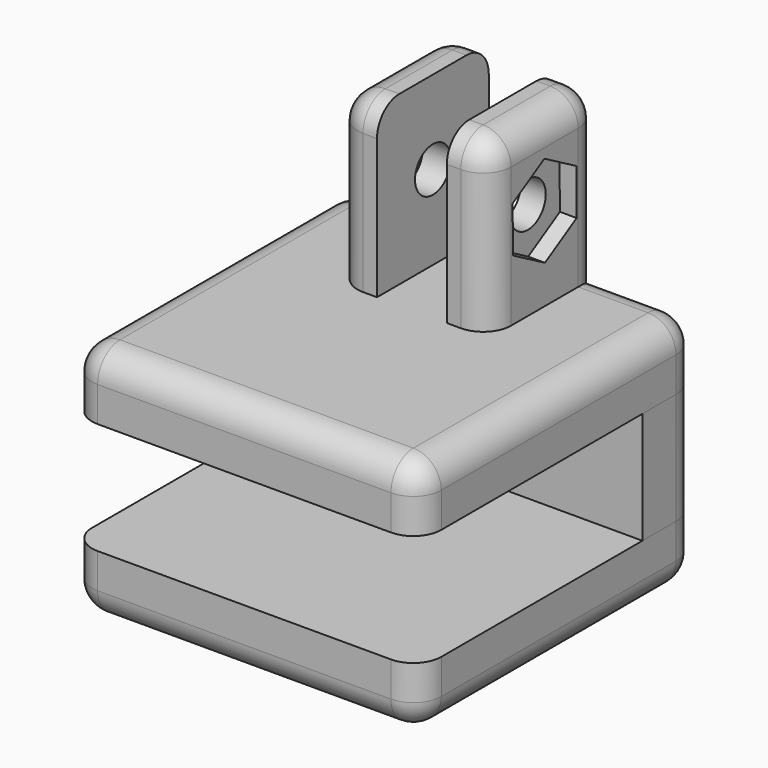
from build123d import *

# Parameters (mm, degrees)
F0_W          = 25
F0_H          = 4.5
F1_DEPTH      = 25
F0_H_2        = 8
F2_DEPTH      = 5
F0_W_2        = 3
F0_H_3        = 12
F3_DEPTH      = 10
F5_DEPTH      = 11.2
F5_DEPTH_BACK = 25
F6_R          = 2
F6_2_R        = 2
F6_3_R        = 2
F7_SIZE       = 1
F9_DEPTH      = 1.2


with BuildPart() as f1:
    # F0 (on Front) → F1 (new body)
    with BuildSketch(Plane.XZ):
        with Locations((0, -6.25)):
            Rectangle(F0_W, F0_H)
    extrude(amount=F1_DEPTH)

    # F6
    f6_edges = [f1.edges().sort_by_distance(p)[0] for p in [
        (12.5, 0, -6.25),
        (-12.5, 0, -6.25),
        (0, 0, -8.5),
        (-12.5, -12.5, -8.5),
        (12.5, -12.5, -8.5),
        (0, -25, -8.5),
        (-12.5, -25, -6.25),
        (12.5, -25, -6.25),
    ]]
    fillet(f6_edges, radius=F6_R)


with BuildPart() as f1b:
    # F0 (on Front) → F1, piece 2 (new body)
    with BuildSketch(Plane.XZ):
        Polygon((12.5, 4), (12.5, 8.5), (5.5, 8.5), (2.5, 8.5), (-2.5, 8.5), (-5.5, 8.5), (-12.5, 8.5), (-12.5, 4), align=None)
    extrude(amount=F1_DEPTH)

    # F0 (on Front) → F3 (join)
    with BuildSketch(Plane.XZ):
        with Locations((4, 14.5)):
            Rectangle(F0_W_2, F0_H_3)
        with Locations((-4, 14.5)):
            Rectangle(F0_W_2, F0_H_3)
    extrude(amount=F3_DEPTH)

    # F4 (on Right) → F5 (cut, two sides)
    with BuildSketch(Plane.YZ) as f5_sk:
        with BuildLine():
            ThreePointArc((-6.6, 14.520585537), (-5, 12.920585537), (-3.4, 14.520585537))
            Line((-3.4, 14.520585537), (-6.6, 14.520585537))
        make_face()
        with BuildLine():
            Line((-6.6, 14.520585537), (-3.4, 14.520585537))
            ThreePointArc((-3.4, 14.520585537), (-5, 16.120585537), (-6.6, 14.520585537))
        make_face()
    extrude(amount=-F5_DEPTH, mode=Mode.SUBTRACT)
    extrude(f5_sk.sketch, amount=F5_DEPTH_BACK, mode=Mode.SUBTRACT)

    # F6#2
    f6_2_edges = [f1b.edges().sort_by_distance(p)[0] for p in [
        (-5.5, -5, 20.5),
        (0, -25, 8.5),
        (12.5, -12.5, 8.5),
        (-12.5, -12.5, 8.5),
        (-12.5, 0, 6.25),
        (-9, 0, 8.5),
        (9, 0, 8.5),
        (12.5, 0, 6.25),
        (-5.5, 0, 14.5),
        (-5.5, -10, 14.5),
        (5.5, 0, 14.5),
        (5.5, -10, 14.5),
        (12.5, -25, 6.25),
        (-12.5, -25, 6.25),
        (5.5, -5, 20.5),
        (4, -10, 20.5),
        (4, 0, 20.5),
        (-4, 0, 20.5),
        (-4, -10, 20.5),
    ]]
    fillet(f6_2_edges, radius=F6_2_R)

    # F7
    f7_edges = [f1b.edges().sort_by_distance(p)[0] for p in [
        (-5.5, -6.6, 14.520586),
    ]]
    chamfer(f7_edges, length=F7_SIZE)

    # F8 (on face) → F9 (cut)
    with BuildSketch(Plane.YZ.offset(5.5)):
        Polygon((-5.0271761454, 17.8113698594), (-7.8634908944, 16.1424424659), (-7.8363147489, 12.8516581434), (-4.9728238546, 11.2298012145), (-2.1365091056, 12.898728608), (-2.1636852511, 16.1895129305), align=None)
    extrude(amount=-F9_DEPTH, mode=Mode.SUBTRACT)


with BuildPart() as f2:
    # F0 (on Front) → F2 (new body)
    with BuildSketch(Plane.XZ):
        Rectangle(F0_W, F0_H_2)
    extrude(amount=F2_DEPTH)

    # F6#3
    f6_3_edges = [f2.edges().sort_by_distance(p)[0] for p in [
        (12.5, 0, 0),
        (-12.5, 0, 0),
    ]]
    fillet(f6_3_edges, radius=F6_3_R)


solid = Compound([f1.part, f1b.part, f2.part])
